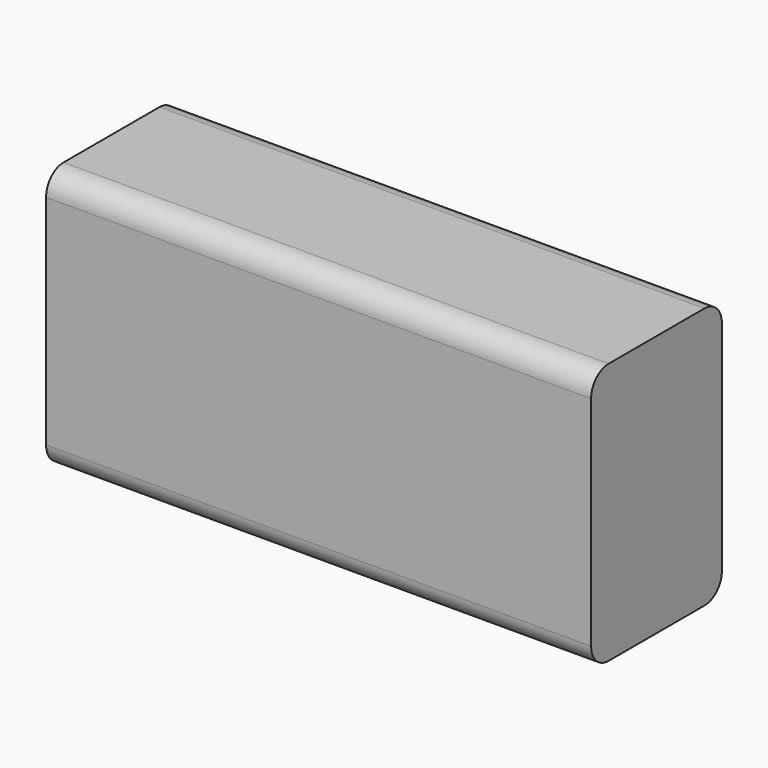
from build123d import *

# Parameters (mm, degrees)
F0_W     = 50
F0_H     = 24
F1_DEPTH = 15
F2_R     = 2
F3_R     = 2
F4_R     = 2


# Not quite as in the source:
# - the program builds the solid bodies; features that only make, move or delete a surface that nothing else refers to are left out


with BuildPart() as f1:
    # F0 (on Front) → F1 (new body)
    with BuildSketch(Plane.XZ):
        Rectangle(F0_W, F0_H)
    extrude(amount=F1_DEPTH)

    # F2
    f2_edges = [f1.edges().sort_by_distance(p)[0] for p in [
        (0, -15, 12),
    ]]
    fillet(f2_edges, radius=F2_R)

    # F3
    f3_edges = [f1.edges().sort_by_distance(p)[0] for p in [
        (0, 0, 12),
        (0, -15, -12),
    ]]
    fillet(f3_edges, radius=F3_R)

    # F4
    f4_edges = [f1.edges().sort_by_distance(p)[0] for p in [
        (0, 0, -12),
    ]]
    fillet(f4_edges, radius=F4_R)


solid = f1.part
